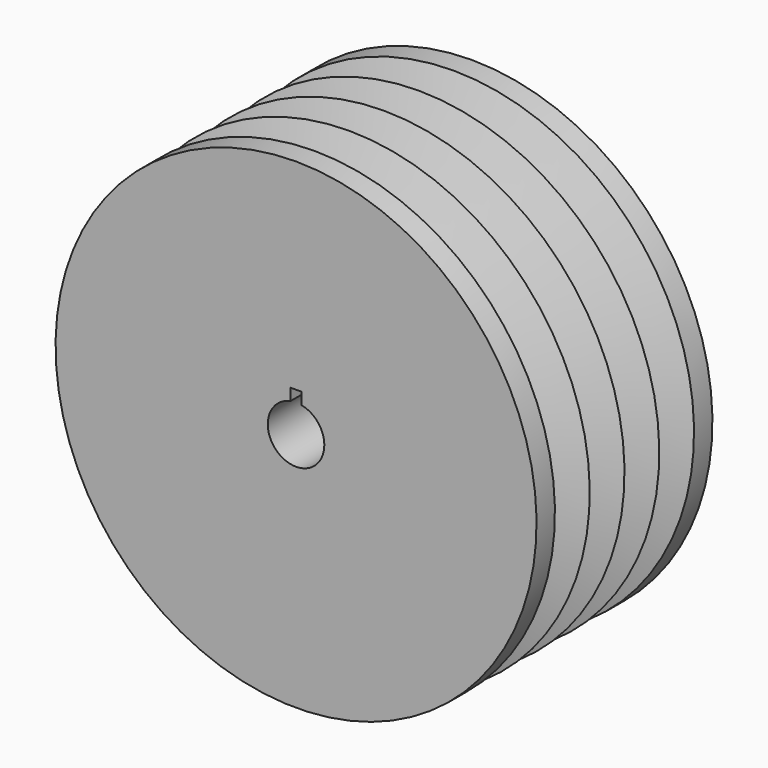
from build123d import *

# Parameters (mm, degrees)
F2_R     = 10
F3_DEPTH = 77.978
F5_DEPTH = 40


# Not quite as in the source:
# - ends of sketch curves that miss each other by under 0.0002 mm in the source are joined


with BuildPart() as f1:
    # F0 (on Right) → F1 (revolve)
    with BuildSketch(Plane.YZ):
        Polygon((-29.7933634734, 31.385529514), (-37.9271134734, 31.385529514), (-37.9271134734, -53.704470486), (-29.7933634734, -53.704470486), (31.7266365266, -53.704470486), (39.8603865266, -53.704470486), (39.8603865266, 31.385529514), (31.7266365266, 31.385529514), (26.815313074, 17.891779514), (21.2579597972, 17.891779514), (16.3466364486, 31.385529514), (11.4353131, 17.891779514), (5.8779598232, 17.891779514), (0.9666364746, 31.385529514), (-3.944686874, 17.891779514), (-9.5020401508, 17.891779514), (-14.4133634994, 31.385529514), (-19.324686848, 17.891779514), (-24.8820401248, 17.891779514), align=None)
    revolve(axis=Axis((0, 0.9666365266, -53.704470486), (0, 1, 0)))

    # F2 (on face) → F3 (cut)
    with BuildSketch(Plane(origin=(0, 39.8603865266, 0), x_dir=(-1, 0, 0), z_dir=(0, 1, 0))):
        with Locations((0, -53.704470486)):
            Circle(F2_R)
    extrude(amount=-F3_DEPTH, mode=Mode.SUBTRACT)

    # F4 (on face) → F5 (cut)
    with BuildSketch(Plane.XZ.offset(37.9271134734)):
        with BuildLine():
            Line((2, -39.704470486), (0, -39.704470486))
            Line((0, -39.704470486), (-2, -39.704470486))
            Line((-2, -39.704470486), (-2, -43.9065115149))
            ThreePointArc((-2, -43.9065115149), (0, -43.704470486), (2, -43.9065115149))
            Line((2, -43.9065115149), (2, -39.704470486))
        make_face()
    extrude(amount=-F5_DEPTH, mode=Mode.SUBTRACT)


solid = f1.part
